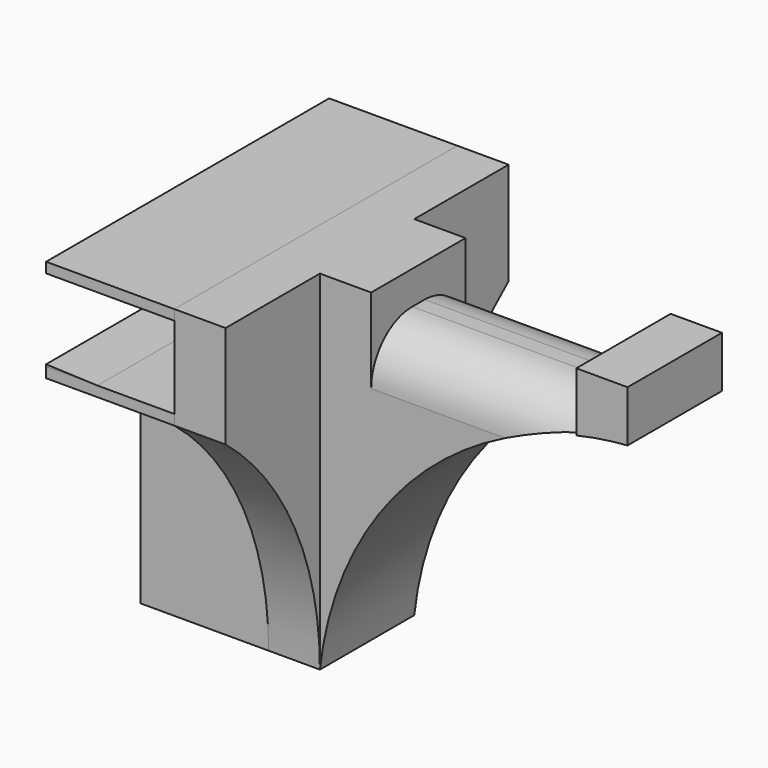
from build123d import *

# Parameters (mm, degrees)
F1_DEPTH     = 25
F2_DEPTH     = 10
F5_DEPTH     = 69
F6_W         = 19
F6_H         = 1.5
F7_DEPTH     = 10
F8_W         = 23
F8_H         = 68
F9_DEPTH     = 100
F10_W        = 40
F10_H        = 6.5
F11_DEPTH    = 46.001
F12_DEPTH    = 23.001
F13_T1_DEPTH = 40


# Not quite as in the source:
# - a fillet or chamfer that OpenCascade refuses, or shapes differently, is made with other operations: its cross-section is extruded or revolved along the edge and cut away or added
# - a feature names something its author has since deleted; it is built from what else it names


with BuildPart() as f1:
    # F0 (on Right) → F1 (new body)
    with BuildSketch(Plane.YZ):
        Polygon((-9.5, -8), (-34.5, -8), (-34.5, -10), (-11.5, -10), (-11.5, -58), (-9.5, -58), align=None)
    extrude(amount=-F1_DEPTH)

    # F10 (on face) → F12 (cut, through all)
    with BuildSketch(Plane.XZ.offset(11.5)):
        with Locations((40, 6.75)):
            Rectangle(F10_W, F10_H)
        with BuildLine():
            Line((110, 10), (70, 10))
            Line((70, 10), (70, 0))
            ThreePointArc((70, 0), (29.5210578409, -18.1597150078), (10, -58))
            Line((10, -58), (110, -58))
            Line((110, -58), (110, 10))
        make_face()
    extrude(amount=F12_DEPTH, mode=Mode.SUBTRACT)


with BuildPart() as f1b:
    # F0 (on Right) → F1, piece 2 (new body)
    with BuildSketch(Plane.YZ):
        Polygon((34.5, -10), (34.5, -8), (9.5, -8), (9.5, -58), (11.5, -58), (11.5, -10), align=None)
    extrude(amount=-F1_DEPTH)


with BuildPart() as f1c:
    # F0 (on Right) → F1, piece 3 (new body)
    with BuildSketch(Plane.YZ):
        Polygon((-9.5, 8), (9.5, 8), (34.5, 8), (34.5, 10), (9.5, 10), (-9.5, 10), (-34.5, 10), (-34.5, 8), align=None)
    extrude(amount=-F1_DEPTH)


with BuildPart() as f2:
    # F0 (on Right) → F2 (new body)
    with BuildSketch(Plane.YZ):
        with BuildLine():
            ThreePointArc((11.5, -58), (17.5468519701, -31.3870332357), (34.5, -10))
            Line((34.5, -10), (11.5, -10))
            Line((11.5, -10), (11.5, -58))
        make_face()
        Polygon((34.5, 8), (9.5, 8), (-9.5, 8), (-34.5, 8), (-34.5, -8), (-9.5, -8), (-9.5, -58), (9.5, -58), (9.5, -8), (34.5, -8), align=None)
        with BuildLine():
            Line((-11.5, -10), (-34.5, -10))
            ThreePointArc((-34.5, -10), (-17.5468519701, -31.3870332357), (-11.5, -58))
            Line((-11.5, -58), (-11.5, -10))
        make_face()
        Polygon((-9.5, -8), (-34.5, -8), (-34.5, -10), (-11.5, -10), (-11.5, -58), (-9.5, -58), align=None)
        Polygon((34.5, -10), (34.5, -8), (9.5, -8), (9.5, -58), (11.5, -58), (11.5, -10), align=None)
        Polygon((-9.5, 8), (9.5, 8), (34.5, 8), (34.5, 10), (9.5, 10), (-9.5, 10), (-34.5, 10), (-34.5, 8), align=None)
    extrude(amount=F2_DEPTH)

    # F8 (on face) → F9 (join)
    with BuildSketch(Plane.YZ.offset(10)):
        with Locations((0, -24)):
            Rectangle(F8_W, F8_H)
    extrude(amount=F9_DEPTH)

    # F10 (on face) → F11 (cut, through all)
    with BuildSketch(Plane.XZ.offset(11.5)):
        with Locations((40, 6.75)):
            Rectangle(F10_W, F10_H)
        with BuildLine():
            Line((110, 10), (70, 10))
            Line((70, 10), (70, 0))
            ThreePointArc((70, 0), (29.5210578409, -18.1597150078), (10, -58))
            Line((10, -58), (110, -58))
            Line((110, -58), (110, 10))
        make_face()
    extrude(amount=-F11_DEPTH, mode=Mode.SUBTRACT)

    # F13: fillet of radius 10 on 2 edges, made by hand

    # F13_s2 → F13_t1 (cut)
    with BuildSketch(Plane.YZ.offset(20)):
        with BuildLine():
            ThreePointArc((11.5, -6.5), (8.5710678119, 0.5710678119), (1.5, 3.5))
            Line((1.5, 3.5), (11.5, 3.5))
            Line((11.5, 3.5), (11.5, -6.5))
        make_face()
        with BuildLine():
            ThreePointArc((-11.5, -6.5), (-8.5710678119, 0.5710678119), (-1.5, 3.5))
            Line((-1.5, 3.5), (-11.5, 3.5))
            Line((-11.5, 3.5), (-11.5, -6.5))
        make_face()
    extrude(amount=F13_T1_DEPTH, mode=Mode.SUBTRACT)


with BuildPart() as f5:
    # F4 (on face) → F5 (new body)
    with BuildSketch(Plane.XZ.offset(34.5)):
        Polygon((-25, -7.6), (-25, -8), (-15, -8), align=None)
    extrude(amount=-F5_DEPTH)

    # F6 (on face) → F7 (cut)
    with BuildSketch(Plane(origin=(-25, 0, 0), x_dir=(0, -1, 0), z_dir=(-1, 0, 0))):
        with Locations((0, -7.25)):
            Rectangle(F6_W, F6_H)
    extrude(amount=-F7_DEPTH, mode=Mode.SUBTRACT)


solid = Compound([f1.part, f1b.part, f1c.part, f2.part, f5.part])
